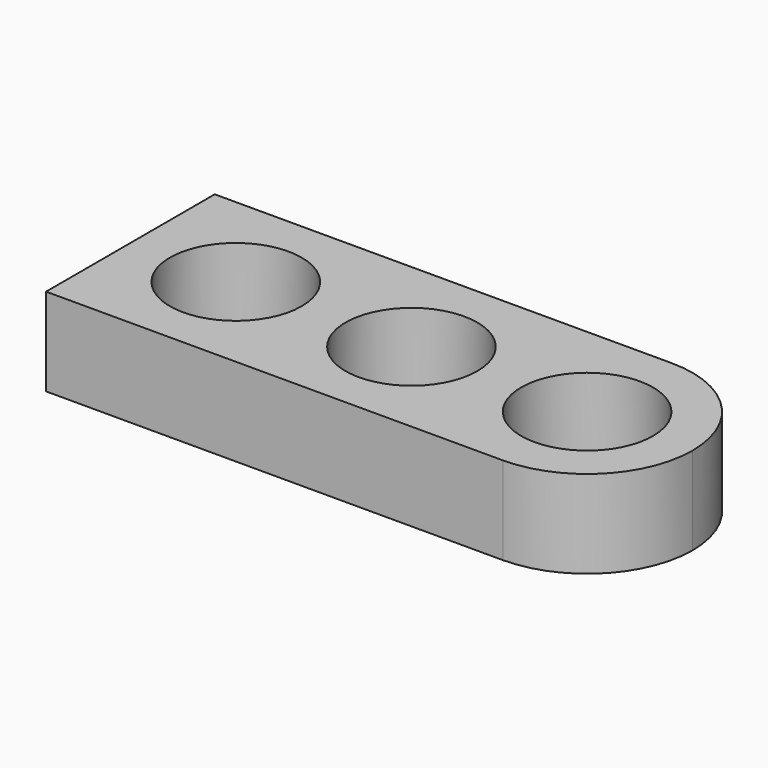
from build123d import *

# Parameters (mm, degrees)
F0_R     = 9.525
F1_DEPTH = 12.7
F2_R     = 15.23999


# Not quite as in the source:
# - a fillet or chamfer is up to 0.001 mm smaller than in the source, because OpenCascade refuses the exact size


with BuildPart() as f1:
    # F0 (on Top) → F1 (new body)
    with BuildSketch(Plane.XY):
        Polygon((-15.24, 0), (0, 0), (0, 30.48), (-81.28, 30.48), (-81.28, 0), align=None)
        with Locations((-66.04, 15.24)):
            Circle(F0_R, mode=Mode.SUBTRACT)
        with Locations((-40.64, 15.24)):
            Circle(F0_R, mode=Mode.SUBTRACT)
        with BuildLine():
            ThreePointArc((-5.715, 15.24), (-8.5048079092, 8.5048079092), (-15.24, 5.715))
            ThreePointArc((-15.24, 5.715), (-21.9751920908, 21.9751920908), (-5.715, 15.24))
        make_face(mode=Mode.SUBTRACT)
    extrude(amount=F1_DEPTH)

    # F2 (radius 15.24 in the source; OpenCascade refuses exactly that, so slightly less here)
    f2_edges = [f1.edges().sort_by_distance(p)[0] for p in [
        (0, 0, 6.35),
        (0, 30.48, 6.35),
    ]]
    fillet(f2_edges, radius=F2_R)


solid = f1.part
